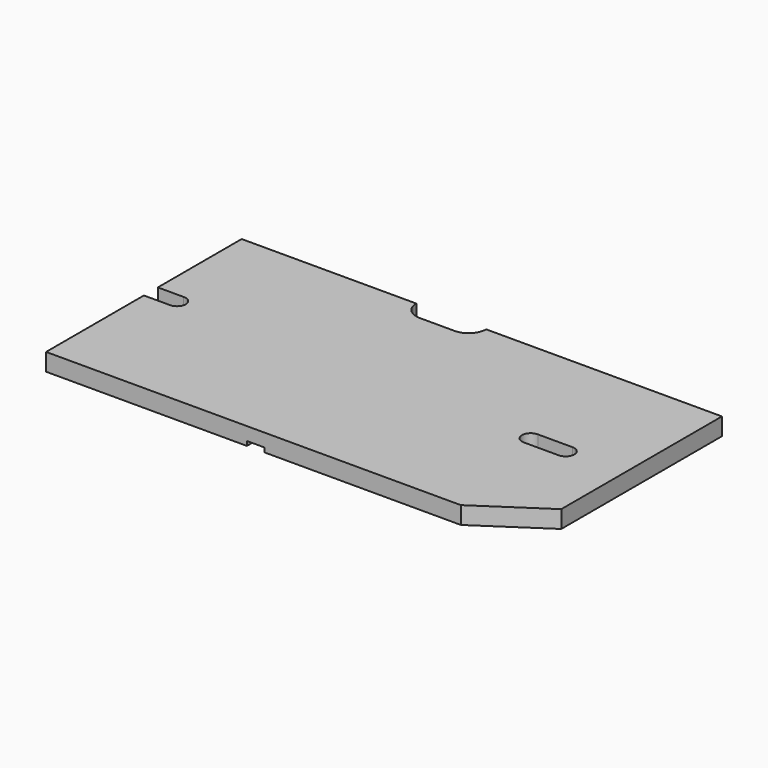
from build123d import *

# Parameters (mm, degrees)
F0_W      = 698.5
F0_H      = 355.6
F1_DEPTH  = 25.4
F3_DEPTH  = 25.401
F4_W      = 88.9
F4_H      = 44.45
F5_DEPTH  = 3.175
F7_DEPTH  = 25.401
F8_W      = 101.6
F8_H      = 25.4
F9_DEPTH  = 25.4
F10_R     = 25.39999
F11_W     = 25.4
F11_H     = 31.75
F12_DEPTH = 6.35


# Not quite as in the source:
# - a fillet or chamfer is up to 0.001 mm smaller than in the source, because OpenCascade refuses the exact size
# - a feature names something its author has since deleted; it is built from what else it names


with BuildPart() as f1:
    # F0 (on Top) → F1 (new body)
    with BuildSketch(Plane.XY):
        Rectangle(F0_W, F0_H)
    extrude(amount=F1_DEPTH)

    # F2 (on face) → F3 (cut, through all)
    with BuildSketch(Plane.XY.offset(25.4)):
        Polygon((349.25, -114.3), (254, -177.8), (349.25, -177.8), align=None)
    extrude(amount=-F3_DEPTH, mode=Mode.SUBTRACT)

    # F4 (on face) → F5 (cut)
    with BuildSketch(Plane(origin=(0, 0, 0), x_dir=(1, 0, 0), z_dir=(0, 0, -1))):
        with Locations((-254, -155.575)):
            Rectangle(F4_W, F4_H)
        with Locations((152.4, -155.575)):
            Rectangle(F4_W, F4_H)
    extrude(amount=-F5_DEPTH, mode=Mode.SUBTRACT)

    # F6 (on face) → F7 (cut, through all)
    with BuildSketch(Plane.XY.offset(25.4)):
        with BuildLine():
            Line((-311.747228622, 0), (-311.747228622, 0.0140503716))
            ThreePointArc((-311.747228622, 0.0140503716), (-298.45, 12.7), (-311.747228622, 25.3859496284))
            Line((-311.747228622, 25.3859496284), (-382.2402954102, 25.3859496284))
            Line((-382.2402954102, 25.3859496284), (-382.2402954102, 0))
            Line((-382.2402954102, 0), (-311.747228622, 0))
        make_face()
        with BuildLine():
            Line((264.16, 12.6990057829), (213.5189091712, 12.6990057829))
            ThreePointArc((213.5189091712, 12.6990057829), (200.66, 0), (213.5189091712, -12.6990057829))
            Line((213.5189091712, -12.6990057829), (213.5189091712, -12.7009942171))
            Line((213.5189091712, -12.7009942171), (264.16, -12.7009942171))
            ThreePointArc((264.16, -12.7009942171), (276.86, -0.0009942171), (264.16, 12.6990057829))
        make_face()
    extrude(amount=-F7_DEPTH, mode=Mode.SUBTRACT)

    # F8 (on face) → F9 (cut)
    with BuildSketch(Plane.XY.offset(25.4)):
        with Locations((-44.45, 165.1)):
            Rectangle(F8_W, F8_H)
    extrude(amount=-F9_DEPTH, mode=Mode.SUBTRACT)

    # F10 (radius 25.4 in the source; OpenCascade refuses exactly that, so slightly less here)
    f10_edges = [f1.edges().sort_by_distance(p)[0] for p in [
        (-95.25, 152.4, 12.7),
        (6.35, 152.4, 12.7),
    ]]
    fillet(f10_edges, radius=F10_R)

    # F11 (on face) → F12 (cut)
    with BuildSketch(Plane(origin=(0, 0, 0), x_dir=(1, 0, 0), z_dir=(0, 0, -1))):
        with Locations((-44.45, 161.925)):
            Rectangle(F11_W, F11_H)
    extrude(amount=-F12_DEPTH, mode=Mode.SUBTRACT)


solid = f1.part
